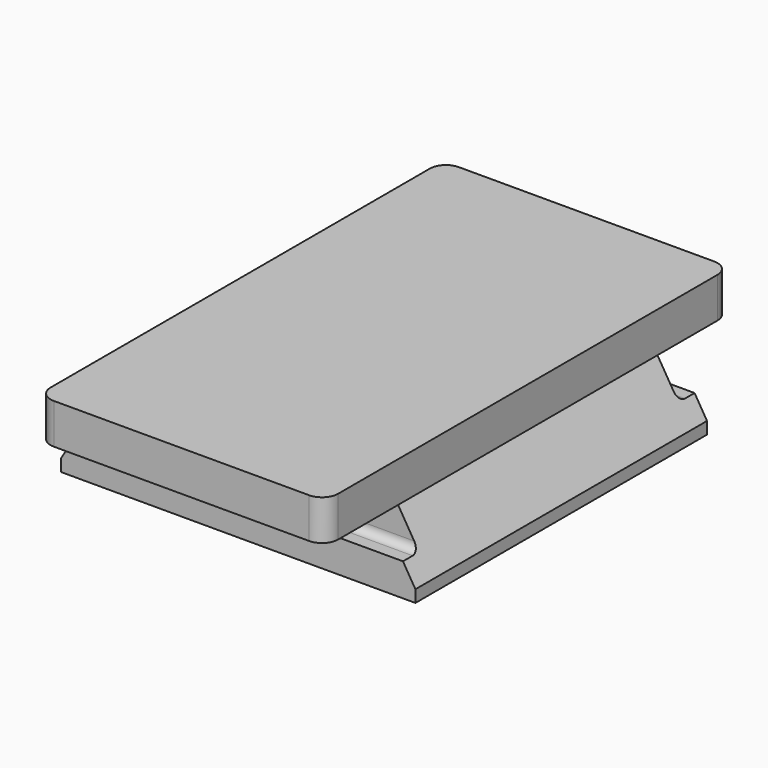
from build123d import *

# Parameters (mm, degrees)
F1_DEPTH = 5
F2_W     = 35.7
F2_H     = 45.25
F4_W     = 44
F4_H     = 45.25
F6_DEPTH = 1.5
F8_DEPTH = 2.5
F9_R     = 1


# Not quite as in the source:
# - a pattern or mirror of a feature is missing from the dataset's text; its kind, count and spacing are read off the source's solid


with BuildPart() as f1:
    # F0 (on Top) → F1 (new body)
    with BuildSketch(Plane.XY):
        with BuildLine():
            Line((-15.85, -31.425), (15.85, -31.425))
            ThreePointArc((15.85, -31.425), (17.2642135624, -30.8392135624), (17.85, -29.425))
            Line((17.85, -29.425), (17.85, 29.425))
            ThreePointArc((17.85, 29.425), (17.2642135624, 30.8392135624), (15.85, 31.425))
            Line((15.85, 31.425), (-15.85, 31.425))
            ThreePointArc((-15.85, 31.425), (-17.2642135624, 30.8392135624), (-17.85, 29.425))
            Line((-17.85, 29.425), (-17.85, -29.425))
            ThreePointArc((-17.85, -29.425), (-17.2642135624, -30.8392135624), (-15.85, -31.425))
        make_face()
    extrude(amount=-F1_DEPTH)

    # F2 (on face) → F5 section 0
    with BuildSketch(Plane(origin=(0, 0, -5), x_dir=(1, 0, 0), z_dir=(0, 0, -1))):
        Rectangle(F2_W, F2_H)
    # F4 (on offset) → F5 section 1
    with BuildSketch(Plane(origin=(0, 0, -11.85), x_dir=(1, 0, 0), z_dir=(0, 0, -1))):
        Rectangle(F4_W, F4_H)
    loft()

    # F4 (on offset) → F6 (join)
    with BuildSketch(Plane(origin=(0, 0, -11.85), x_dir=(1, 0, 0), z_dir=(0, 0, -1))):
        Rectangle(F4_W, F4_H)
    extrude(amount=F6_DEPTH)

    # F7 (on face) → F8 (cut)
    with BuildSketch(Plane.XZ.offset(22.625)):
        Polygon((5.9, -5), (0, -5), (-5.9, -5), (-5.9, -9.3), (0, -9.3), (5.9, -9.3), align=None)
        Polygon((-7.6, -9.3), (-7.6, -5), (-17.85, -5), (-20.4551094891, -9.3), align=None)
        Polygon((17.85, -5), (7.6, -5), (7.6, -9.3), (20.4551094891, -9.3), align=None)
    f8 = extrude(amount=-F8_DEPTH, mode=Mode.SUBTRACT)

    # F8_copies: F8 across plane
    add(f8.mirror(Plane.ZX), mode=Mode.SUBTRACT)

    # F9
    f9_edges = [f1.edges().sort_by_distance(p)[0] for p in [
        (-14.027555, -20.125, -9.3),
        (0, -20.125, -9.3),
        (14.027555, -20.125, -9.3),
        (14.027555, 20.125, -9.3),
        (0, 20.125, -9.3),
        (-14.027555, 20.125, -9.3),
    ]]
    fillet(f9_edges, radius=F9_R)


solid = f1.part
